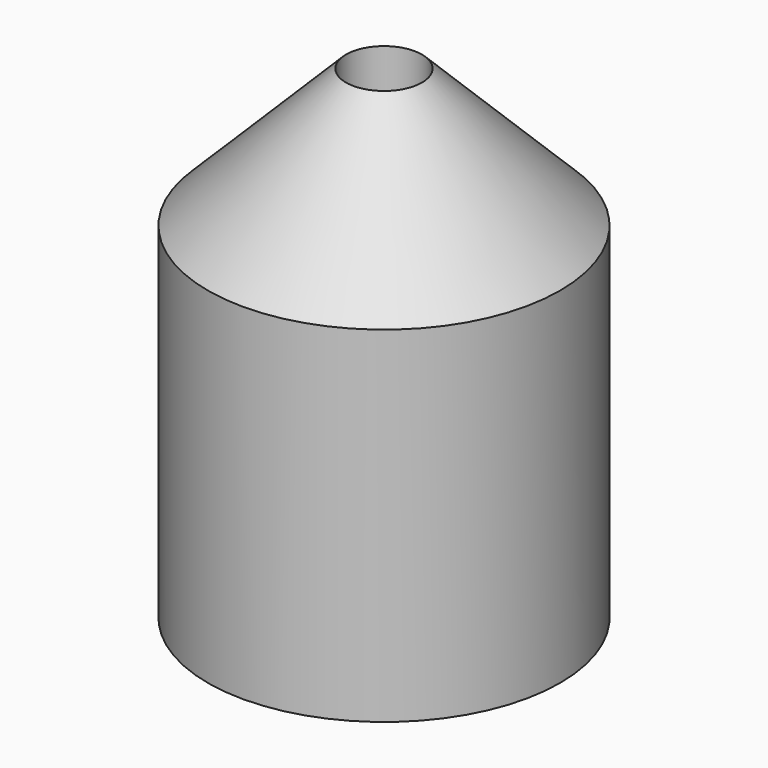
from build123d import *

# Parameters (mm, degrees)
F0_R     = 25.5
F0_R_2   = 5.5
F1_DEPTH = 70
F2_SIZE  = 19.99999


# Not quite as in the source:
# - a fillet or chamfer is up to 0.001 mm smaller than in the source, because OpenCascade refuses the exact size


with BuildPart() as f1:
    # F0 (on Top) → F1 (new body)
    with BuildSketch(Plane.XY):
        Circle(F0_R)
        Circle(F0_R_2, mode=Mode.SUBTRACT)
    extrude(amount=F1_DEPTH)

    # F2 (size 20 in the source; OpenCascade refuses exactly that, so slightly less here)
    f2_edges = [f1.edges().sort_by_distance(p)[0] for p in [
        (-25.5, 0, 70),
    ]]
    chamfer(f2_edges, length=F2_SIZE)


solid = f1.part
